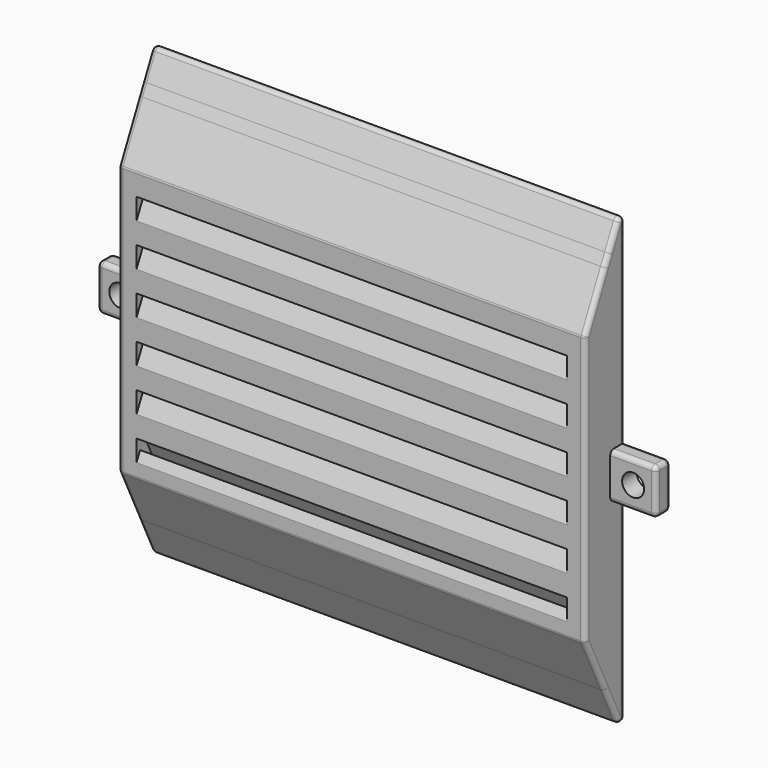
from build123d import *

# Parameters (mm, degrees)
F1_DEPTH = 51
F2_DEPTH = 49
F3_DEPTH = 2
F5_W     = 5
F5_H     = 5
F5_R     = 1.2
F6_DEPTH = 2
F7_R     = 0.5
F8_R     = 0.49999


# Not quite as in the source:
# - a fillet or chamfer is up to 0.001 mm smaller than in the source, because OpenCascade refuses the exact size
# - a feature names something its author has since deleted; it is built from what else it names


with BuildPart() as f1:
    # F0 (on Right) → F1 (new body)
    with BuildSketch(Plane.YZ):
        Polygon((1.6229308846, 40.6768469676), (-1.0759725176, 35.0152704514), (-1.0759725176, 32.6913771026), (1.6229308846, 38.3529536188), align=None)
        Polygon((1.6229308846, 38.3529536188), (-1.0759725176, 32.6913771026), (-1.0759725176, 30.3674837537), (1.6229308846, 36.0290602699), (4.3218342869, 30.3674837537), (4.3218342869, 32.6913771026), (2.6721461458, 36.1519810022), (2.1768369961, 37.1910069443), (2.7307431076, 38.3529536188), (4.3218342869, 35.0152704514), (4.3218342869, 37.3391638002), (3.284649219, 39.5149002932), (3.8385553305, 40.6768469676), (4.3218342869, 39.6630571491), (4.3218342869, 41.9869504979), (3.8385553305, 43.0007403164), align=None)
        Polygon((2.1768369961, 41.838793642), (1.6229308846, 40.6768469676), (1.6229308846, 38.3529536188), (3.8385553305, 43.0007403164), (4.3218342869, 41.9869504979), (4.3218342869, 46.3384234838), align=None)
        Polygon((1.6229308846, 36.0290602699), (-1.0759725176, 30.3674837537), (-1.0759725176, 28.0435904049), (1.6229308846, 33.7051669211), align=None)
        Polygon((1.6229308846, 33.7051669211), (-1.0759725176, 28.0435904049), (-1.0759725176, 25.7196970561), (1.6229308846, 31.3812735723), (4.3218342869, 25.7196970561), (4.3218342869, 28.0435904049), align=None)
        Polygon((4.3218342869, 30.3674837537), (1.6229308846, 36.0290602699), (1.6229308846, 33.7051669211), (4.3218342869, 28.0435904049), align=None)
        Polygon((1.6229308846, 31.3812735723), (-1.0759725176, 25.7196970561), (-1.0759725176, 23.3958037072), (1.6229308846, 29.0573802234), align=None)
        Polygon((1.6229308846, 29.0573802234), (-1.0759725176, 23.3958037072), (-1.0759725176, 21.0719103584), (1.6229308846, 26.7334868746), (4.3218342869, 21.0719103584), (4.3218342869, 23.3958037072), align=None)
        Polygon((4.3218342869, 25.7196970561), (1.6229308846, 31.3812735723), (1.6229308846, 29.0573802234), (4.3218342869, 23.3958037072), align=None)
        Polygon((2.6721461458, 36.1519810022), (4.3218342869, 32.6913771026), (4.3218342869, 34.3225207567), (4.3218342869, 35.0152704514), (2.7307431076, 38.3529536188), (2.1768369961, 37.1910069443), align=None)
        Polygon((4.3218342869, 37.3391638002), (4.3218342869, 39.6630571491), (3.8385553305, 40.6768469676), (3.284649219, 39.5149002932), align=None)
        Polygon((1.6229308846, 26.7334868746), (-1.0759725176, 21.0719103584), (-1.0759725176, 18.7480170096), (1.6229308846, 24.4095935257), align=None)
        Polygon((1.6229308846, 24.4095935257), (-1.0759725176, 18.7480170096), (-1.0759725176, 16.4241236607), (1.6229308846, 22.0857001769), (4.3218342869, 16.4241236607), (4.3218342869, 18.7480170096), align=None)
        Polygon((4.3218342869, 21.0719103584), (1.6229308846, 26.7334868746), (1.6229308846, 24.4095935257), (4.3218342869, 18.7480170096), align=None)
        Polygon((1.6229308846, 22.0857001769), (-1.0759725176, 16.4241236607), (-1.0759725176, 14.1002303119), (1.6229308846, 19.7618068281), align=None)
        Polygon((1.6229308846, 19.7618068281), (-1.0759725176, 14.1002303119), (-1.0759725176, 11.776336963), (1.6229308846, 17.4379134792), (4.3218342869, 11.776336963), (4.3218342869, 14.1002303119), align=None)
        Polygon((4.3218342869, 16.4241236607), (1.6229308846, 22.0857001769), (1.6229308846, 19.7618068281), (4.3218342869, 14.1002303119), align=None)
        Polygon((1.6229308846, 17.4379134792), (-1.0759725176, 11.776336963), (-1.0759725176, 9.4524436142), (1.6229308846, 15.1140201304), align=None)
        Polygon((1.6229308846, 15.1140201304), (-1.0759725176, 9.4524436142), (-1.0759725176, 7.1285502654), (-0.5926935612, 8.1423400839), (1.6229308846, 3.4945533862), (4.3218342869, -2.16702313), (4.3218342869, 0.1568702189), (1.6229308846, 5.8184467351), (-0.0387874498, 9.3042867583), (0.5151186617, 10.4662334327), (1.6229308846, 8.1423400839), (4.3218342869, 2.4807635677), (4.3218342869, 4.8046569165), (3.4631130188, 6.6060241537), (1.6229308846, 10.4662334327), (1.0690247732, 11.6281801071), (1.6229308846, 12.7901267816), (4.3218342869, 7.1285502654), (4.3218342869, 9.4524436142), align=None)
        Polygon((4.3218342869, 11.776336963), (1.6229308846, 17.4379134792), (1.6229308846, 15.1140201304), (4.3218342869, 9.4524436142), align=None)
        Polygon((-0.5926935612, 8.1423400839), (-1.0759725176, 7.1285502654), (-1.0759725176, 5.6615765162), (1.6229308846, 0), (1.6229308846, 1.6931712119), (1.6229308846, 3.4945533862), align=None)
        Polygon((1.6229308846, 1.6931712119), (1.6229308846, 0), (4.3218342869, -5.6615765162), (4.3218342869, -2.16702313), (1.6229308846, 3.4945533862), align=None)
        Polygon((4.3218342869, 6.559693444), (4.3218342869, 7.1285502654), (1.6229308846, 12.7901267816), (1.6229308846, 11.0159027272), (1.6229308846, 10.4662334327), (3.4631130188, 6.6060241537), align=None)
        Polygon((4.3218342869, 5.354326211), (4.3218342869, 6.559693444), (3.4631130188, 6.6060241537), (4.3218342869, 4.8046569165), align=None)
        Polygon((1.6229308846, 5.8184467351), (4.3218342869, 0.1568702189), (4.3218342869, 2.4807635677), (1.6229308846, 8.1423400839), align=None)
        Polygon((1.6229308846, 11.0159027272), (1.6229308846, 12.7901267816), (1.0690247732, 11.6281801071), (1.6229308846, 10.4662334327), align=None)
        Polygon((-0.0387874498, 9.3042867583), (1.6229308846, 5.8184467351), (1.6229308846, 8.1423400839), (0.5151186617, 10.4662334327), align=None)
    extrude(amount=-F1_DEPTH)

    # F0 (on Right) → F2 (cut)
    with BuildSketch(Plane.YZ):
        Polygon((1.6229308846, 38.3529536188), (-1.0759725176, 32.6913771026), (-1.0759725176, 30.3674837537), (1.6229308846, 36.0290602699), (4.3218342869, 30.3674837537), (4.3218342869, 32.6913771026), (2.6721461458, 36.1519810022), (2.1768369961, 37.1910069443), (2.7307431076, 38.3529536188), (4.3218342869, 35.0152704514), (4.3218342869, 37.3391638002), (3.284649219, 39.5149002932), (3.8385553305, 40.6768469676), (4.3218342869, 39.6630571491), (4.3218342869, 41.9869504979), (3.8385553305, 43.0007403164), align=None)
        Polygon((1.6229308846, 33.7051669211), (-1.0759725176, 28.0435904049), (-1.0759725176, 25.7196970561), (1.6229308846, 31.3812735723), (4.3218342869, 25.7196970561), (4.3218342869, 28.0435904049), align=None)
        Polygon((1.6229308846, 29.0573802234), (-1.0759725176, 23.3958037072), (-1.0759725176, 21.0719103584), (1.6229308846, 26.7334868746), (4.3218342869, 21.0719103584), (4.3218342869, 23.3958037072), align=None)
        Polygon((1.6229308846, 24.4095935257), (-1.0759725176, 18.7480170096), (-1.0759725176, 16.4241236607), (1.6229308846, 22.0857001769), (4.3218342869, 16.4241236607), (4.3218342869, 18.7480170096), align=None)
        Polygon((1.6229308846, 19.7618068281), (-1.0759725176, 14.1002303119), (-1.0759725176, 11.776336963), (1.6229308846, 17.4379134792), (4.3218342869, 11.776336963), (4.3218342869, 14.1002303119), align=None)
        Polygon((1.6229308846, 15.1140201304), (-1.0759725176, 9.4524436142), (-1.0759725176, 7.1285502654), (-0.5926935612, 8.1423400839), (1.6229308846, 3.4945533862), (4.3218342869, -2.16702313), (4.3218342869, 0.1568702189), (1.6229308846, 5.8184467351), (-0.0387874498, 9.3042867583), (0.5151186617, 10.4662334327), (1.6229308846, 8.1423400839), (4.3218342869, 2.4807635677), (4.3218342869, 4.8046569165), (3.4631130188, 6.6060241537), (1.6229308846, 10.4662334327), (1.0690247732, 11.6281801071), (1.6229308846, 12.7901267816), (4.3218342869, 7.1285502654), (4.3218342869, 9.4524436142), align=None)
    extrude(amount=-F2_DEPTH, mode=Mode.SUBTRACT)

    # F0 (on Right) → F3 (join)
    with BuildSketch(Plane.YZ):
        Polygon((1.6229308846, 40.6768469676), (-1.0759725176, 35.0152704514), (-1.0759725176, 32.6913771026), (1.6229308846, 38.3529536188), align=None)
        Polygon((1.6229308846, 38.3529536188), (-1.0759725176, 32.6913771026), (-1.0759725176, 30.3674837537), (1.6229308846, 36.0290602699), (4.3218342869, 30.3674837537), (4.3218342869, 32.6913771026), (2.6721461458, 36.1519810022), (2.1768369961, 37.1910069443), (2.7307431076, 38.3529536188), (4.3218342869, 35.0152704514), (4.3218342869, 37.3391638002), (3.284649219, 39.5149002932), (3.8385553305, 40.6768469676), (4.3218342869, 39.6630571491), (4.3218342869, 41.9869504979), (3.8385553305, 43.0007403164), align=None)
        Polygon((2.1768369961, 41.838793642), (1.6229308846, 40.6768469676), (1.6229308846, 38.3529536188), (3.8385553305, 43.0007403164), (4.3218342869, 41.9869504979), (4.3218342869, 46.3384234838), align=None)
        Polygon((1.6229308846, 36.0290602699), (-1.0759725176, 30.3674837537), (-1.0759725176, 28.0435904049), (1.6229308846, 33.7051669211), align=None)
        Polygon((1.6229308846, 33.7051669211), (-1.0759725176, 28.0435904049), (-1.0759725176, 25.7196970561), (1.6229308846, 31.3812735723), (4.3218342869, 25.7196970561), (4.3218342869, 28.0435904049), align=None)
        Polygon((4.3218342869, 30.3674837537), (1.6229308846, 36.0290602699), (1.6229308846, 33.7051669211), (4.3218342869, 28.0435904049), align=None)
        Polygon((1.6229308846, 31.3812735723), (-1.0759725176, 25.7196970561), (-1.0759725176, 23.3958037072), (1.6229308846, 29.0573802234), align=None)
        Polygon((1.6229308846, 29.0573802234), (-1.0759725176, 23.3958037072), (-1.0759725176, 21.0719103584), (1.6229308846, 26.7334868746), (4.3218342869, 21.0719103584), (4.3218342869, 23.3958037072), align=None)
        Polygon((4.3218342869, 25.7196970561), (1.6229308846, 31.3812735723), (1.6229308846, 29.0573802234), (4.3218342869, 23.3958037072), align=None)
        Polygon((2.6721461458, 36.1519810022), (4.3218342869, 32.6913771026), (4.3218342869, 34.3225207567), (4.3218342869, 35.0152704514), (2.7307431076, 38.3529536188), (2.1768369961, 37.1910069443), align=None)
        Polygon((4.3218342869, 37.3391638002), (4.3218342869, 39.6630571491), (3.8385553305, 40.6768469676), (3.284649219, 39.5149002932), align=None)
        Polygon((1.6229308846, 26.7334868746), (-1.0759725176, 21.0719103584), (-1.0759725176, 18.7480170096), (1.6229308846, 24.4095935257), align=None)
        Polygon((1.6229308846, 24.4095935257), (-1.0759725176, 18.7480170096), (-1.0759725176, 16.4241236607), (1.6229308846, 22.0857001769), (4.3218342869, 16.4241236607), (4.3218342869, 18.7480170096), align=None)
        Polygon((4.3218342869, 21.0719103584), (1.6229308846, 26.7334868746), (1.6229308846, 24.4095935257), (4.3218342869, 18.7480170096), align=None)
        Polygon((1.6229308846, 22.0857001769), (-1.0759725176, 16.4241236607), (-1.0759725176, 14.1002303119), (1.6229308846, 19.7618068281), align=None)
        Polygon((1.6229308846, 19.7618068281), (-1.0759725176, 14.1002303119), (-1.0759725176, 11.776336963), (1.6229308846, 17.4379134792), (4.3218342869, 11.776336963), (4.3218342869, 14.1002303119), align=None)
        Polygon((4.3218342869, 16.4241236607), (1.6229308846, 22.0857001769), (1.6229308846, 19.7618068281), (4.3218342869, 14.1002303119), align=None)
        Polygon((1.6229308846, 17.4379134792), (-1.0759725176, 11.776336963), (-1.0759725176, 9.4524436142), (1.6229308846, 15.1140201304), align=None)
        Polygon((1.6229308846, 15.1140201304), (-1.0759725176, 9.4524436142), (-1.0759725176, 7.1285502654), (-0.5926935612, 8.1423400839), (1.6229308846, 3.4945533862), (4.3218342869, -2.16702313), (4.3218342869, 0.1568702189), (1.6229308846, 5.8184467351), (-0.0387874498, 9.3042867583), (0.5151186617, 10.4662334327), (1.6229308846, 8.1423400839), (4.3218342869, 2.4807635677), (4.3218342869, 4.8046569165), (3.4631130188, 6.6060241537), (1.6229308846, 10.4662334327), (1.0690247732, 11.6281801071), (1.6229308846, 12.7901267816), (4.3218342869, 7.1285502654), (4.3218342869, 9.4524436142), align=None)
        Polygon((4.3218342869, 11.776336963), (1.6229308846, 17.4379134792), (1.6229308846, 15.1140201304), (4.3218342869, 9.4524436142), align=None)
        Polygon((-0.5926935612, 8.1423400839), (-1.0759725176, 7.1285502654), (-1.0759725176, 5.6615765162), (1.6229308846, 0), (1.6229308846, 1.6931712119), (1.6229308846, 3.4945533862), align=None)
        Polygon((1.6229308846, 1.6931712119), (1.6229308846, 0), (4.3218342869, -5.6615765162), (4.3218342869, -2.16702313), (1.6229308846, 3.4945533862), align=None)
        Polygon((4.3218342869, 6.559693444), (4.3218342869, 7.1285502654), (1.6229308846, 12.7901267816), (1.6229308846, 11.0159027272), (1.6229308846, 10.4662334327), (3.4631130188, 6.6060241537), align=None)
        Polygon((4.3218342869, 5.354326211), (4.3218342869, 6.559693444), (3.4631130188, 6.6060241537), (4.3218342869, 4.8046569165), align=None)
        Polygon((1.6229308846, 5.8184467351), (4.3218342869, 0.1568702189), (4.3218342869, 2.4807635677), (1.6229308846, 8.1423400839), align=None)
    extrude(amount=-F3_DEPTH)

    # F5 (on plane+point) → F6 (join)
    with BuildSketch(Plane.XZ.offset(-4.3218342869)):
        with Locations((-53.5, 20.3384234838)):
            Rectangle(F5_W, F5_H)
        with Locations((-53.5, 20.3384234838)):
            Circle(F5_R, mode=Mode.SUBTRACT)
        with Locations((2.5, 20.3384234838)):
            Rectangle(F5_W, F5_H)
        with Locations((2.5, 20.3384234838)):
            Circle(F5_R, mode=Mode.SUBTRACT)
    extrude(amount=F6_DEPTH)

    # F7
    f7_edges = [f1.edges().sort_by_distance(p)[0] for p in [
        (-53.5, 2.321834, 22.838423),
        (-53.5, 4.321834, 22.838423),
        (-56, 3.321834, 22.838423),
        (-56, 3.321834, 17.838423),
        (-56, 2.321834, 20.338423),
        (-56, 4.321834, 20.338423),
        (-53.5, 2.321834, 17.838423),
        (-53.5, 4.321834, 17.838423),
        (2.5, 4.321834, 17.838423),
        (2.5, 4.321834, 22.838423),
        (5, 4.321834, 20.338423),
        (2.5, 2.321834, 17.838423),
        (5, 3.321834, 22.838423),
        (5, 3.321834, 17.838423),
        (5, 2.321834, 20.338423),
        (2.5, 2.321834, 22.838423),
    ]]
    fillet(f7_edges, radius=F7_R)

    # F8 (radius 0.5 in the source; OpenCascade refuses exactly that, so slightly less here)
    f8_edges = [f1.edges().sort_by_distance(p)[0] for p in [
        (-25.5, 4.321834, 46.338423),
        (-25.5, 4.321834, -5.661577),
        (-25.5, -1.075973, 5.661577),
        (-25.5, -1.075973, 35.01527),
        (-51, 1.622931, 40.676847),
        (0, 1.622931, 40.676847),
        (0, -1.075973, 20.338423),
        (-51, -1.075973, 20.338423),
        (-51, 1.622931, 0),
        (0, 1.622931, 0),
        (-51, 4.321834, 34.588423),
        (-51, 4.321834, 6.088423),
        (0, 4.321834, 34.588423),
        (0, 4.321834, 6.088423),
    ]]
    fillet(f8_edges, radius=F8_R)


solid = f1.part
